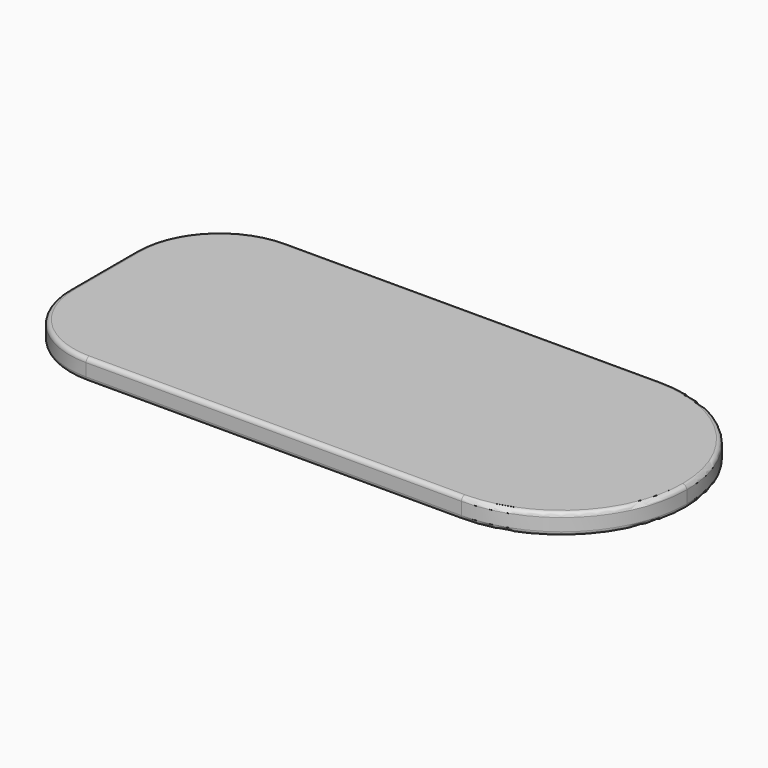
from build123d import *

# Parameters (mm, degrees)
F0_W     = 355.6
F0_H     = 152.4
F1_DEPTH = 12.7
F2_R     = 76.2
F3_R     = 76.19999
F4_R     = 50.8
F5_R     = 50.8
F6_R     = 2.54


# Not quite as in the source:
# - a fillet or chamfer is up to 0.001 mm smaller than in the source, because OpenCascade refuses the exact size


with BuildPart() as f1:
    # F0 (on Top) → F1 (new body)
    with BuildSketch(Plane.XY):
        Rectangle(F0_W, F0_H)
    extrude(amount=F1_DEPTH)

    # F2
    f2_edges = [f1.edges().sort_by_distance(p)[0] for p in [
        (177.8, 76.2, 6.35),
    ]]
    fillet(f2_edges, radius=F2_R)

    # F3 (radius 76.2 in the source; OpenCascade refuses exactly that, so slightly less here)
    f3_edges = [f1.edges().sort_by_distance(p)[0] for p in [
        (177.8, -76.2, 6.35),
    ]]
    fillet(f3_edges, radius=F3_R)

    # F4
    f4_edges = [f1.edges().sort_by_distance(p)[0] for p in [
        (-177.8, 76.2, 6.35),
    ]]
    fillet(f4_edges, radius=F4_R)

    # F5
    f5_edges = [f1.edges().sort_by_distance(p)[0] for p in [
        (-177.8, -76.2, 6.35),
    ]]
    fillet(f5_edges, radius=F5_R)

    # F6
    f6_edges = [f1.edges().sort_by_distance(p)[0] for p in [
        (-12.7, 76.2, 12.7),
        (-12.7, 76.2, 0),
    ]]
    fillet(f6_edges, radius=F6_R)


solid = f1.part
